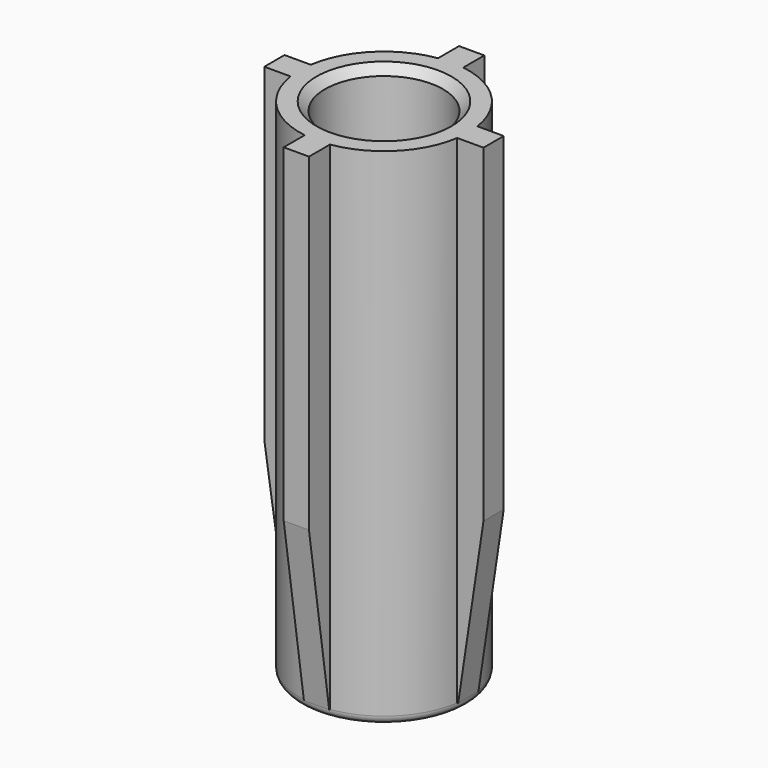
from build123d import *

# Parameters (mm, degrees)
F1_R        = 5
F1_R_2      = 3.5
F2_DEPTH    = 30
F4_W        = 1.5
F4_H        = 2.639524132
F5_DEPTH    = 29.5
F6_COUNT    = 4
F8_R        = 3.5
F8_R_2      = 1.5
F9_DEPTH    = 1.5
F10_SIZE2   = 1.49999
F10_SIZE    = 9.99999
F10_2_SIZE2 = 1.49999
F10_2_SIZE  = 9.99999
F10_3_SIZE2 = 1.49999
F10_3_SIZE  = 9.99999
F10_4_SIZE2 = 1.49999
F10_4_SIZE  = 9.99999
F11_SIZE    = 0.5
F12_R       = 0.49999


# Not quite as in the source:
# - a fillet or chamfer is up to 0.001 mm smaller than in the source, because OpenCascade refuses the exact size


with BuildPart() as f2:
    # F1 (on offset) → F2 (new body)
    with BuildSketch(Plane.XY):
        with Locations((-25, 25)):
            Circle(F1_R)
        with Locations((-25, 25)):
            Circle(F1_R_2, mode=Mode.SUBTRACT)
    extrude(amount=-F2_DEPTH)

    # F4 (on offset) → F5 (join)
    with BuildSketch(Plane.XY):
        with Locations((-25, 30.180237934)):
            Rectangle(F4_W, F4_H)
    extrude(amount=-F5_DEPTH)

    # F6: F2 ×4 about axis
    f6_axis = Axis((-25, 25, 0), (0, 0, 1))


with BuildPart() as f2_1:
    add(f2.part)
    for i in range(1, F6_COUNT):
        add(f2.part.rotate(f6_axis, i * 360 / F6_COUNT))

    # F8 (on offset) → F9 (join)
    with BuildSketch(Plane.XY.offset(-30)):
        with Locations((-25, 25)):
            Circle(F8_R)
        with Locations((-25, 25)):
            Circle(F8_R_2, mode=Mode.SUBTRACT)
    extrude(amount=F9_DEPTH)

    # F10 (size 10 and 1.5 in the source; OpenCascade refuses exactly that, so slightly less here)
    f10_edges = [f2_1.edges().sort_by_distance(p)[0] for p in [
        (-25, 18.5, -29.5),
    ]]
    f10_side = f2_1.faces().sort_by_distance((-25, 18.5, -14.75))[0]
    chamfer(f10_edges, length=F10_SIZE, length2=F10_SIZE2, reference=f10_side)

    # F10#2 (size 10 and 1.5 in the source; OpenCascade refuses exactly that, so slightly less here)
    f10_2_edges = [f2_1.edges().sort_by_distance(p)[0] for p in [
        (-18.5, 25, -29.5),
    ]]
    f10_2_side = f2_1.faces().sort_by_distance((-18.5, 25, -14.75))[0]
    chamfer(f10_2_edges, length=F10_2_SIZE, length2=F10_2_SIZE2, reference=f10_2_side)

    # F10#3 (size 10 and 1.5 in the source; OpenCascade refuses exactly that, so slightly less here)
    f10_3_edges = [f2_1.edges().sort_by_distance(p)[0] for p in [
        (-25, 31.5, -29.5),
    ]]
    f10_3_side = f2_1.faces().sort_by_distance((-25, 31.5, -14.75))[0]
    chamfer(f10_3_edges, length=F10_3_SIZE, length2=F10_3_SIZE2, reference=f10_3_side)

    # F10#4 (size 10 and 1.5 in the source; OpenCascade refuses exactly that, so slightly less here)
    f10_4_edges = [f2_1.edges().sort_by_distance(p)[0] for p in [
        (-31.5, 25, -29.5),
    ]]
    f10_4_side = f2_1.faces().sort_by_distance((-31.5, 25, -14.75))[0]
    chamfer(f10_4_edges, length=F10_4_SIZE, length2=F10_4_SIZE2, reference=f10_4_side)

    # F11
    f11_edges = [f2_1.edges().sort_by_distance(p)[0] for p in [
        (-28.5, 25, 0),
        (-26.5, 25, -28.5),
    ]]
    chamfer(f11_edges, length=F11_SIZE)

    # F12 (radius 0.5 in the source; OpenCascade refuses exactly that, so slightly less here)
    f12_edges = [f2_1.edges().sort_by_distance(p)[0] for p in [
        (-30, 25, -30),
    ]]
    fillet(f12_edges, radius=F12_R)


solid = f2_1.part
